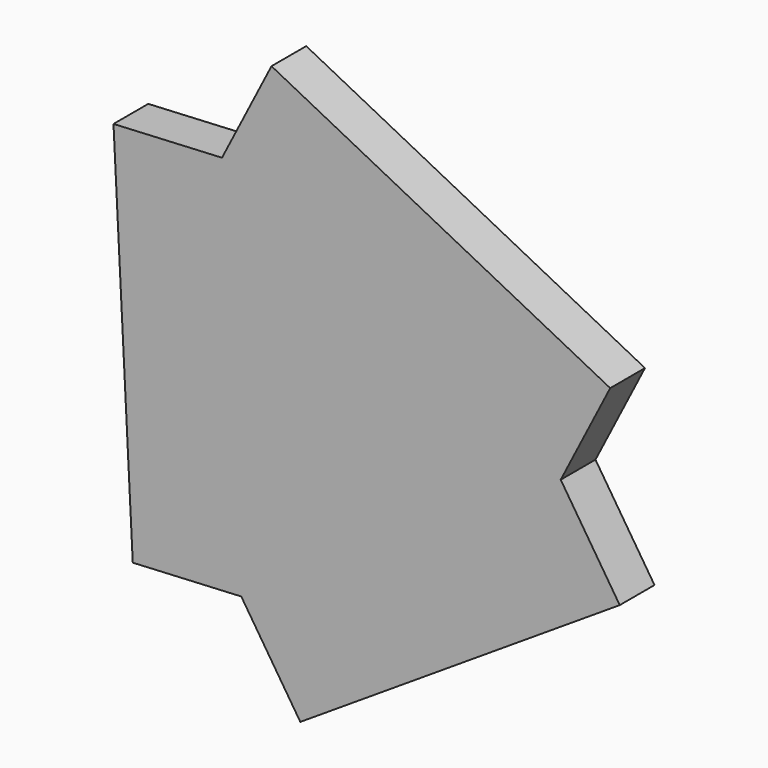
from build123d import *

# Parameters (mm, degrees)
F2_DEPTH = 5.08
F3_DEPTH = 12.7
F4_DEPTH = 12.7
F5_DEPTH = 12.7


# Not quite as in the source:
# - the program builds the solid bodies; features that only make, move or delete a surface that nothing else refers to are left out


with BuildPart() as f2:
    # F1 (on Front) → F2 (new body)
    with BuildSketch(Plane.XZ):
        Polygon((39.5757543065, 1.3013935037), (-0.0187108435, 21.5584816091), (2.2353688255, -22.8598751128), align=None)
    extrude(amount=F2_DEPTH)

    # F3 (add): a face of the model
    f3_faces = [f2.faces().sort_by_distance(p)[0] for p in [
        (1.108328991, -2.54, -0.6506967518),
    ]]
    extrude(f3_faces, amount=F3_DEPTH)

    # F4 (add): a face of the model
    f4_faces = [f2.faces().sort_by_distance(p)[0] for p in [
        (20.905561566, -2.54, -10.7792408046),
    ]]
    extrude(f4_faces, amount=F4_DEPTH)

    # F5 (add): a face of the model
    f5_faces = [f2.faces().sort_by_distance(p)[0] for p in [
        (19.7785217315, -2.54, 11.4299375564),
    ]]
    extrude(f5_faces, amount=F5_DEPTH)


solid = f2.part
